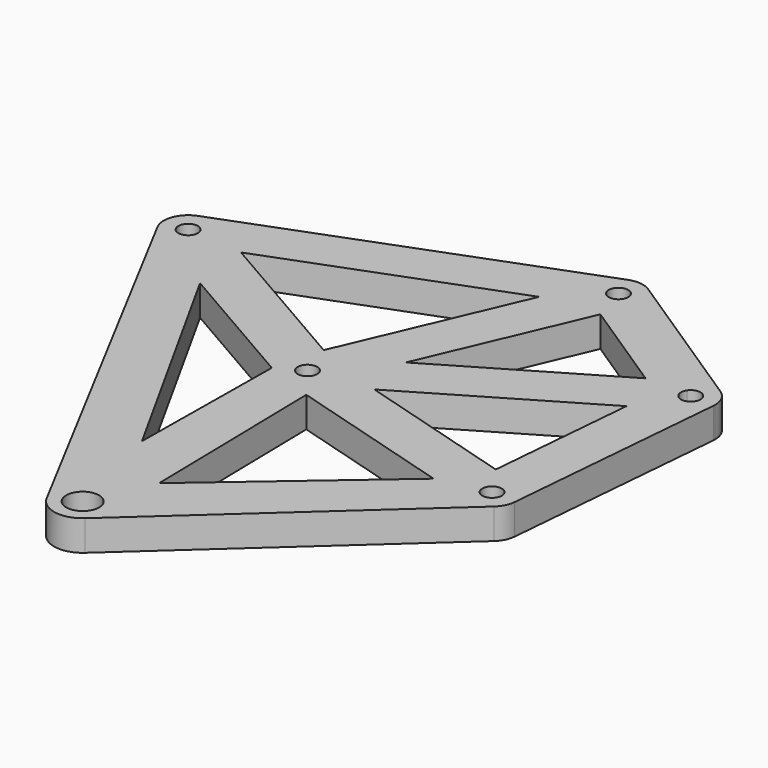
from build123d import *

# Parameters (mm, degrees)
F1_R     = 0.8
F1_R_2   = 1.35
F2_DEPTH = 2.5


# Not quite as in the source:
# - a feature of the source that left no trace in its solid (it failed there, or was rolled back) is left out


with BuildPart() as f2:
    # F1 (on Top) → F2 (new body)
    with BuildSketch(Plane.XY):
        with BuildLine():
            ThreePointArc((5.199444907, 41.7323711721), (4.3598959993, 41.9935980712), (3.4894439174, 41.8695213434))
            ThreePointArc((3.4894439174, 41.8695213434), (2.3279381226, 40.7038354404), (2.4337804668, 39.0616671377))
            ThreePointArc((2.4337804668, 39.0616671377), (2.7613029651, 38.610701313), (3.200555093, 38.2676288279))
            ThreePointArc((3.200555093, 38.2676288279), (4.1741960688, 38.0001664676), (5.1544139045, 38.2424181103))
            ThreePointArc((5.1544139045, 38.2424181103), (5.9188408607, 38.9774609565), (6.2, 40))
            ThreePointArc((6.2, 40), (6.1361812507, 40.5012007226), (5.9487978357, 40.9704154419))
            ThreePointArc((5.9487978357, 40.9704154419), (5.625957109, 41.402371678), (5.199444907, 41.7323711721))
        make_face()
        with Locations((4.2, 40)):
            Circle(F1_R, mode=Mode.SUBTRACT)
        with BuildLine():
            Line((27.6104340169, 46.7612620152), (29.4612530015, 51.0867715523))
            ThreePointArc((29.4612530015, 51.0867715523), (29.9151450158, 51.7429749383), (30.5894439174, 52.1695213434))
            Line((30.5894439174, 52.1695213434), (3.4894439174, 41.8695213434))
            ThreePointArc((3.4894439174, 41.8695213434), (4.3598959993, 41.9935980712), (5.199444907, 41.7323711721))
            Line((5.199444907, 41.7323711721), (8.8310911779, 39.6371906312))
            Line((8.8310911779, 39.6371906312), (27.6104340169, 46.7612620152))
        make_face()
        with BuildLine():
            ThreePointArc((32.009384409, 48.4300337542), (32.5519790638, 48.74033708), (32.972287567, 49.202979356))
            ThreePointArc((32.972287567, 49.202979356), (33.0623576694, 49.3544337965), (33.1387469985, 49.5132284477))
            ThreePointArc((33.1387469985, 49.5132284477), (33.2592720583, 49.8984368026), (33.3, 50.3))
            ThreePointArc((33.3, 50.3), (33.0598354025, 51.2502522592), (32.397020644, 51.972287567))
            ThreePointArc((32.397020644, 51.972287567), (31.5169424001, 52.2881991839), (30.5894439174, 52.1695213434))
            ThreePointArc((30.5894439174, 52.1695213434), (29.9151450158, 51.7429749383), (29.4612530015, 51.0867715523))
            ThreePointArc((29.4612530015, 51.0867715523), (29.3852086666, 49.7224412157), (30.202979356, 48.627712433))
            ThreePointArc((30.202979356, 48.627712433), (31.0824346588, 48.311868887), (32.009384409, 48.4300337542))
        make_face()
        with BuildLine():
            ThreePointArc((31.9689150268, 49.8611917424), (30.5334714547, 50.5289846922), (32.1, 50.3))
            ThreePointArc((32.1, 50.3), (32.0665285453, 50.0710153078), (31.9689150268, 49.8611917424))
        make_face(mode=Mode.SUBTRACT)
        with BuildLine():
            ThreePointArc((20.1501364504, 6.325323864), (20.2166788322, 5.7441722888), (20.4246920484, 5.1974588868))
            ThreePointArc((20.4246920484, 5.1974588868), (22.0958795292, 3.985008284), (24.0790139172, 4.5595359673))
            ThreePointArc((24.0790139172, 4.5595359673), (24.6486254566, 5.3482076659), (24.85, 6.3))
            ThreePointArc((24.85, 6.3), (24.8498894798, 6.3227910674), (24.8495579296, 6.3455799911))
            ThreePointArc((24.8495579296, 6.3455799911), (24.7691945263, 6.9109469713), (24.5548374569, 7.4402381443))
            ThreePointArc((24.5548374569, 7.4402381443), (22.9138153936, 8.6132783706), (20.9678942394, 8.0818956025))
            ThreePointArc((20.9678942394, 8.0818956025), (20.3695522772, 7.2918127346), (20.1501364504, 6.325323864))
        make_face()
        with Locations((22.5, 6.3)):
            Circle(F1_R_2, mode=Mode.SUBTRACT)
        with BuildLine():
            ThreePointArc((44.2, 23.7), (43.800697674, 24.8990692042), (42.7622330434, 25.6193472862))
            ThreePointArc((42.7622330434, 25.6193472862), (41.7779870797, 25.6549693336), (40.8960802037, 25.2165068958))
            ThreePointArc((40.8960802037, 25.2165068958), (40.4202125368, 24.6123357857), (40.2075188236, 23.8732592327))
            ThreePointArc((40.2075188236, 23.8732592327), (40.548821119, 22.571457443), (41.6377669566, 21.7806527138))
            ThreePointArc((41.6377669566, 21.7806527138), (42.6480080175, 21.7508235544), (43.5438416317, 22.2187540147))
            ThreePointArc((43.5438416317, 22.2187540147), (43.991778392, 22.8114448842), (44.1924811764, 23.5267407673))
            ThreePointArc((44.1924811764, 23.5267407673), (44.1981194099, 23.6132888496), (44.2, 23.7))
        make_face()
        with Locations((42.2, 23.7)):
            Circle(F1_R, mode=Mode.SUBTRACT)
        with BuildLine():
            ThreePointArc((42.7852559244, 43.8234542237), (42.4204567714, 43.5480540323), (42.127712433, 43.197020644))
            ThreePointArc((42.127712433, 43.197020644), (41.9102999519, 42.7550066627), (41.8075188236, 42.2732592327))
            ThreePointArc((41.8075188236, 42.2732592327), (42.0006206287, 41.2269399345), (42.702979356, 40.427712433))
            ThreePointArc((42.702979356, 40.427712433), (43.7515555461, 40.1005868024), (44.8147440756, 40.3765457763))
            ThreePointArc((44.8147440756, 40.3765457763), (45.4916344335, 41.0330543859), (45.7924811764, 41.9267407673))
            ThreePointArc((45.7924811764, 41.9267407673), (45.7981194099, 42.0132888496), (45.8, 42.1))
            ThreePointArc((45.8, 42.1), (45.5598354025, 43.0502522592), (44.897020644, 43.772287567))
            ThreePointArc((44.897020644, 43.772287567), (43.8484444539, 44.0994131976), (42.7852559244, 43.8234542237))
        make_face()
        with BuildLine():
            ThreePointArc((44.6, 42.1), (43.5710153078, 41.3334714547), (43.1310849732, 42.5388082576))
            ThreePointArc((43.1310849732, 42.5388082576), (44.0289846922, 42.8665285453), (44.6, 42.1))
        make_face(mode=Mode.SUBTRACT)
        with BuildLine():
            ThreePointArc((22.9622330434, 31.4193472862), (22.1534536929, 31.4847455551), (21.3852559244, 31.2234542237))
            ThreePointArc((21.3852559244, 31.2234542237), (20.8983520938, 30.8210047561), (20.5612530015, 30.2867715523))
            ThreePointArc((20.5612530015, 30.2867715523), (20.4429200591, 29.9121141894), (20.400116128, 29.5215522247))
            ThreePointArc((20.400116128, 29.5215522247), (20.6627449521, 28.5090686712), (21.400555093, 27.7676288279))
            ThreePointArc((21.400555093, 27.7676288279), (21.6135843834, 27.6611007428), (21.8377669566, 27.5806527138))
            ThreePointArc((21.8377669566, 27.5806527138), (22.6465463071, 27.5152544449), (23.4147440756, 27.7765457763))
            ThreePointArc((23.4147440756, 27.7765457763), (23.9016479062, 28.1789952439), (24.2387469985, 28.7132284477))
            ThreePointArc((24.2387469985, 28.7132284477), (24.3592720583, 29.0984368026), (24.4, 29.5))
            ThreePointArc((24.4, 29.5), (24.3999059403, 29.5193966531), (24.3996237698, 29.5387914818))
            ThreePointArc((24.3996237698, 29.5387914818), (24.1221080901, 30.5170269053), (23.399444907, 31.2323711721))
            ThreePointArc((23.399444907, 31.2323711721), (23.1864156166, 31.3388992572), (22.9622330434, 31.4193472862))
        make_face()
        with Locations((22.4, 29.5)):
            Circle(F1_R, mode=Mode.SUBTRACT)
        with BuildLine():
            Line((41.6377669566, 21.7806527138), (38.1039741935, 22.8158041293))
            Line((38.1039741935, 22.8158041293), (24.7527433965, 11.336176711))
            Line((24.7527433965, 11.336176711), (24.8495579296, 6.3455799911))
            ThreePointArc((24.8495579296, 6.3455799911), (24.8498894798, 6.3227910674), (24.85, 6.3))
            ThreePointArc((24.85, 6.3), (24.6486254566, 5.3482076659), (24.0790139172, 4.5595359673))
            Line((24.0790139172, 4.5595359673), (43.5438416317, 22.2187540147))
            ThreePointArc((43.5438416317, 22.2187540147), (42.6480080175, 21.7508235544), (41.6377669566, 21.7806527138))
        make_face()
        with BuildLine():
            Line((44.8147440756, 40.3765457763), (41.4714130157, 38.408042442))
            Line((41.4714130157, 38.408042442), (40.4190386777, 26.3057375549))
            Line((40.4190386777, 26.3057375549), (42.7622330434, 25.6193472862))
            ThreePointArc((42.7622330434, 25.6193472862), (43.800697674, 24.8990692042), (44.2, 23.7))
            ThreePointArc((44.2, 23.7), (44.1981194099, 23.6132888496), (44.1924811764, 23.5267407673))
            Line((44.1924811764, 23.5267407673), (45.7924811764, 41.9267407673))
            ThreePointArc((45.7924811764, 41.9267407673), (45.4916344335, 41.0330543859), (44.8147440756, 40.3765457763))
        make_face()
        with BuildLine():
            Line((24.8495579296, 6.3455799911), (24.7527433965, 11.336176711))
            Line((24.7527433965, 11.336176711), (23.1551857529, 9.9625680299))
            Line((23.1551857529, 9.9625680299), (24.5548374569, 7.4402381443))
            ThreePointArc((24.5548374569, 7.4402381443), (24.7691945263, 6.9109469713), (24.8495579296, 6.3455799911))
        make_face()
        with BuildLine():
            Line((24.5548374569, 7.4402381443), (23.1551857529, 9.9625680299))
            Line((23.1551857529, 9.9625680299), (20.9678942394, 8.0818956025))
            ThreePointArc((20.9678942394, 8.0818956025), (22.9138153936, 8.6132783706), (24.5548374569, 7.4402381443))
        make_face()
        with BuildLine():
            Line((40.2075188236, 23.8732592327), (40.2781200828, 24.6851737134))
            Line((40.2781200828, 24.6851737134), (38.1039741935, 22.8158041293))
            Line((38.1039741935, 22.8158041293), (41.6377669566, 21.7806527138))
            ThreePointArc((41.6377669566, 21.7806527138), (40.548821119, 22.571457443), (40.2075188236, 23.8732592327))
        make_face()
        with BuildLine():
            Line((42.7622330434, 25.6193472862), (40.4190386777, 26.3057375549))
            Line((40.4190386777, 26.3057375549), (40.2781200828, 24.6851737134))
            Line((40.2781200828, 24.6851737134), (40.8960802037, 25.2165068958))
            ThreePointArc((40.8960802037, 25.2165068958), (41.7779870797, 25.6549693336), (42.7622330434, 25.6193472862))
        make_face()
        with BuildLine():
            Line((42.702979356, 40.427712433), (41.7040205766, 41.0830293923))
            Line((41.7040205766, 41.0830293923), (41.4714130157, 38.408042442))
            Line((41.4714130157, 38.408042442), (44.8147440756, 40.3765457763))
            ThreePointArc((44.8147440756, 40.3765457763), (43.7515555461, 40.1005868024), (42.702979356, 40.427712433))
        make_face()
        with BuildLine():
            ThreePointArc((42.702979356, 40.427712433), (42.0006206287, 41.2269399345), (41.8075188236, 42.2732592327))
            Line((41.8075188236, 42.2732592327), (41.7040205766, 41.0830293923))
            Line((41.7040205766, 41.0830293923), (42.702979356, 40.427712433))
        make_face()
        with BuildLine():
            Line((40.8960802037, 25.2165068958), (40.2781200828, 24.6851737134))
            Line((40.2781200828, 24.6851737134), (40.2075188236, 23.8732592327))
            ThreePointArc((40.2075188236, 23.8732592327), (40.4202125368, 24.6123357857), (40.8960802037, 25.2165068958))
        make_face()
        with BuildLine():
            ThreePointArc((3.200555093, 38.2676288279), (2.7613029651, 38.610701313), (2.4337804668, 39.0616671377))
            Line((2.4337804668, 39.0616671377), (20.4246920484, 5.1974588868))
            ThreePointArc((20.4246920484, 5.1974588868), (20.2166788322, 5.7441722888), (20.1501364504, 6.325323864))
            Line((20.1501364504, 6.325323864), (20.2458362488, 15.2055432508))
            Line((20.2458362488, 15.2055432508), (9.4489187614, 34.6628036346))
            Line((9.4489187614, 34.6628036346), (3.200555093, 38.2676288279))
        make_face()
        with BuildLine():
            Line((23.1551857529, 9.9625680299), (20.2458362488, 15.2055432508))
            Line((20.2458362488, 15.2055432508), (20.1501364504, 6.325323864))
            ThreePointArc((20.1501364504, 6.325323864), (20.3695522772, 7.2918127346), (20.9678942394, 8.0818956025))
            Line((20.9678942394, 8.0818956025), (23.1551857529, 9.9625680299))
        make_face()
        with BuildLine():
            Line((24.7527433965, 11.336176711), (24.452468903, 26.8147299215))
            Line((24.452468903, 26.8147299215), (21.8377669566, 27.5806527138))
            ThreePointArc((21.8377669566, 27.5806527138), (21.6135843834, 27.6611007428), (21.400555093, 27.7676288279))
            Line((21.400555093, 27.7676288279), (20.3875129911, 28.3520761944))
            Line((20.3875129911, 28.3520761944), (20.2458362488, 15.2055432508))
            Line((20.2458362488, 15.2055432508), (23.1551857529, 9.9625680299))
            Line((23.1551857529, 9.9625680299), (24.7527433965, 11.336176711))
        make_face()
        with BuildLine():
            Line((33.1387469985, 49.5132284477), (32.9986081891, 49.185713028))
            Line((32.9986081891, 49.185713028), (41.9354850239, 43.3231218243))
            Line((41.9354850239, 43.3231218243), (42.7852559244, 43.8234542237))
            ThreePointArc((42.7852559244, 43.8234542237), (43.8484444539, 44.0994131976), (44.897020644, 43.772287567))
            Line((44.897020644, 43.772287567), (32.397020644, 51.972287567))
            ThreePointArc((32.397020644, 51.972287567), (33.0598354025, 51.2502522592), (33.3, 50.3))
            ThreePointArc((33.3, 50.3), (33.2592720583, 49.8984368026), (33.1387469985, 49.5132284477))
        make_face()
        Polygon((41.9354850239, 43.3231218243), (32.9986081891, 49.185713028), (32.1994534098, 47.3180254538), (40.0139218466, 42.1917341592), align=None)
        with BuildLine():
            Line((42.127712433, 43.197020644), (41.9354850239, 43.3231218243))
            Line((41.9354850239, 43.3231218243), (40.0139218466, 42.1917341592))
            Line((40.0139218466, 42.1917341592), (41.7040205766, 41.0830293923))
            Line((41.7040205766, 41.0830293923), (41.8075188236, 42.2732592327))
            ThreePointArc((41.8075188236, 42.2732592327), (41.9102999519, 42.7550066627), (42.127712433, 43.197020644))
        make_face()
        with BuildLine():
            Line((42.7852559244, 43.8234542237), (41.9354850239, 43.3231218243))
            Line((41.9354850239, 43.3231218243), (42.127712433, 43.197020644))
            ThreePointArc((42.127712433, 43.197020644), (42.4204567714, 43.5480540323), (42.7852559244, 43.8234542237))
        make_face()
        with BuildLine():
            Line((32.9986081891, 49.185713028), (32.972287567, 49.202979356))
            ThreePointArc((32.972287567, 49.202979356), (32.5519790638, 48.74033708), (32.009384409, 48.4300337542))
            Line((32.009384409, 48.4300337542), (31.0557778484, 48.068276622))
            Line((31.0557778484, 48.068276622), (32.1994534098, 47.3180254538))
            Line((32.1994534098, 47.3180254538), (32.9986081891, 49.185713028))
        make_face()
        with BuildLine():
            ThreePointArc((33.1387469985, 49.5132284477), (33.0623576694, 49.3544337965), (32.972287567, 49.202979356))
            Line((32.972287567, 49.202979356), (32.9986081891, 49.185713028))
            Line((32.9986081891, 49.185713028), (33.1387469985, 49.5132284477))
        make_face()
        with BuildLine():
            Line((31.0557778484, 48.068276622), (32.009384409, 48.4300337542))
            ThreePointArc((32.009384409, 48.4300337542), (31.0824346588, 48.311868887), (30.202979356, 48.627712433))
            Line((30.202979356, 48.627712433), (31.0557778484, 48.068276622))
        make_face()
        with BuildLine():
            Line((31.0557778484, 48.068276622), (30.202979356, 48.627712433))
            ThreePointArc((30.202979356, 48.627712433), (29.3852086666, 49.7224412157), (29.4612530015, 51.0867715523))
            Line((29.4612530015, 51.0867715523), (27.6104340169, 46.7612620152))
            Line((27.6104340169, 46.7612620152), (31.0557778484, 48.068276622))
        make_face()
        with BuildLine():
            Line((7.0611867859, 38.9657653668), (8.8310911779, 39.6371906312))
            Line((8.8310911779, 39.6371906312), (5.199444907, 41.7323711721))
            ThreePointArc((5.199444907, 41.7323711721), (5.625957109, 41.402371678), (5.9487978357, 40.9704154419))
            Line((5.9487978357, 40.9704154419), (7.0611867859, 38.9657653668))
        make_face()
        with BuildLine():
            Line((5.1544139045, 38.2424181103), (7.0611867859, 38.9657653668))
            Line((7.0611867859, 38.9657653668), (5.9487978357, 40.9704154419))
            ThreePointArc((5.9487978357, 40.9704154419), (6.1361812507, 40.5012007226), (6.2, 40))
            ThreePointArc((6.2, 40), (5.9188408607, 38.9774609565), (5.1544139045, 38.2424181103))
        make_face()
        with BuildLine():
            Line((9.4489187614, 34.6628036346), (7.0611867859, 38.9657653668))
            Line((7.0611867859, 38.9657653668), (5.1544139045, 38.2424181103))
            ThreePointArc((5.1544139045, 38.2424181103), (4.1741960688, 38.0001664676), (3.200555093, 38.2676288279))
            Line((3.200555093, 38.2676288279), (9.4489187614, 34.6628036346))
        make_face()
        with BuildLine():
            Line((20.5612530015, 30.2867715523), (21.4476690943, 32.3583956794))
            Line((21.4476690943, 32.3583956794), (8.8310911779, 39.6371906312))
            Line((8.8310911779, 39.6371906312), (7.0611867859, 38.9657653668))
            Line((7.0611867859, 38.9657653668), (9.4489187614, 34.6628036346))
            Line((9.4489187614, 34.6628036346), (20.3875129911, 28.3520761944))
            Line((20.3875129911, 28.3520761944), (20.400116128, 29.5215522247))
            ThreePointArc((20.400116128, 29.5215522247), (20.4429200591, 29.9121141894), (20.5612530015, 30.2867715523))
        make_face()
        with BuildLine():
            Line((21.3852559244, 31.2234542237), (22.3897518441, 31.8148864007))
            Line((22.3897518441, 31.8148864007), (21.4476690943, 32.3583956794))
            Line((21.4476690943, 32.3583956794), (20.5612530015, 30.2867715523))
            ThreePointArc((20.5612530015, 30.2867715523), (20.8983520938, 30.8210047561), (21.3852559244, 31.2234542237))
        make_face()
        Polygon((26.6355518827, 34.3147499748), (32.1994534098, 47.3180254538), (31.0557778484, 48.068276622), (27.6104340169, 46.7612620152), (21.4476690943, 32.3583956794), (22.3897518441, 31.8148864007), align=None)
        Polygon((25.1255087716, 30.7856604567), (26.6355518827, 34.3147499748), (22.3897518441, 31.8148864007), (23.1920320855, 31.3520324152), align=None)
        Polygon((40.4190386777, 26.3057375549), (27.3959062448, 30.1205945302), (24.4223018654, 28.3697807367), (24.452468903, 26.8147299215), (38.1039741935, 22.8158041293), (40.2781200828, 24.6851737134), align=None)
        Polygon((27.3959062448, 30.1205945302), (25.1255087716, 30.7856604567), (24.4079671049, 29.1087091458), (24.4223018654, 28.3697807367), align=None)
        with BuildLine():
            ThreePointArc((21.400555093, 27.7676288279), (20.6627449521, 28.5090686712), (20.400116128, 29.5215522247))
            Line((20.400116128, 29.5215522247), (20.3875129911, 28.3520761944))
            Line((20.3875129911, 28.3520761944), (21.400555093, 27.7676288279))
        make_face()
        with BuildLine():
            Line((24.452468903, 26.8147299215), (24.4223018654, 28.3697807367))
            Line((24.4223018654, 28.3697807367), (23.4147440756, 27.7765457763))
            ThreePointArc((23.4147440756, 27.7765457763), (22.6465463071, 27.5152544449), (21.8377669566, 27.5806527138))
            Line((21.8377669566, 27.5806527138), (24.452468903, 26.8147299215))
        make_face()
        with BuildLine():
            Line((24.4223018654, 28.3697807367), (24.4079671049, 29.1087091458))
            Line((24.4079671049, 29.1087091458), (24.2387469985, 28.7132284477))
            ThreePointArc((24.2387469985, 28.7132284477), (23.9016479062, 28.1789952439), (23.4147440756, 27.7765457763))
            Line((23.4147440756, 27.7765457763), (24.4223018654, 28.3697807367))
        make_face()
        with BuildLine():
            Line((24.2387469985, 28.7132284477), (24.4079671049, 29.1087091458))
            Line((24.4079671049, 29.1087091458), (24.3996237698, 29.5387914818))
            ThreePointArc((24.3996237698, 29.5387914818), (24.3999059403, 29.5193966531), (24.4, 29.5))
            ThreePointArc((24.4, 29.5), (24.3592720583, 29.0984368026), (24.2387469985, 28.7132284477))
        make_face()
        with BuildLine():
            Line((24.4079671049, 29.1087091458), (25.1255087716, 30.7856604567))
            Line((25.1255087716, 30.7856604567), (23.1920320855, 31.3520324152))
            Line((23.1920320855, 31.3520324152), (23.399444907, 31.2323711721))
            ThreePointArc((23.399444907, 31.2323711721), (24.1221080901, 30.5170269053), (24.3996237698, 29.5387914818))
            Line((24.3996237698, 29.5387914818), (24.4079671049, 29.1087091458))
        make_face()
        with BuildLine():
            Line((23.1920320855, 31.3520324152), (22.3897518441, 31.8148864007))
            Line((22.3897518441, 31.8148864007), (21.3852559244, 31.2234542237))
            ThreePointArc((21.3852559244, 31.2234542237), (22.1534536929, 31.4847455551), (22.9622330434, 31.4193472862))
            Line((22.9622330434, 31.4193472862), (23.1920320855, 31.3520324152))
        make_face()
        with BuildLine():
            Line((23.399444907, 31.2323711721), (23.1920320855, 31.3520324152))
            Line((23.1920320855, 31.3520324152), (22.9622330434, 31.4193472862))
            ThreePointArc((22.9622330434, 31.4193472862), (23.1864156166, 31.3388992572), (23.399444907, 31.2323711721))
        make_face()
        Polygon((41.7040205766, 41.0830293923), (40.0139218466, 42.1917341592), (26.6355518827, 34.3147499748), (25.1255087716, 30.7856604567), (27.3959062448, 30.1205945302), (41.4714130157, 38.408042442), align=None)
    extrude(amount=-F2_DEPTH)


solid = f2.part
